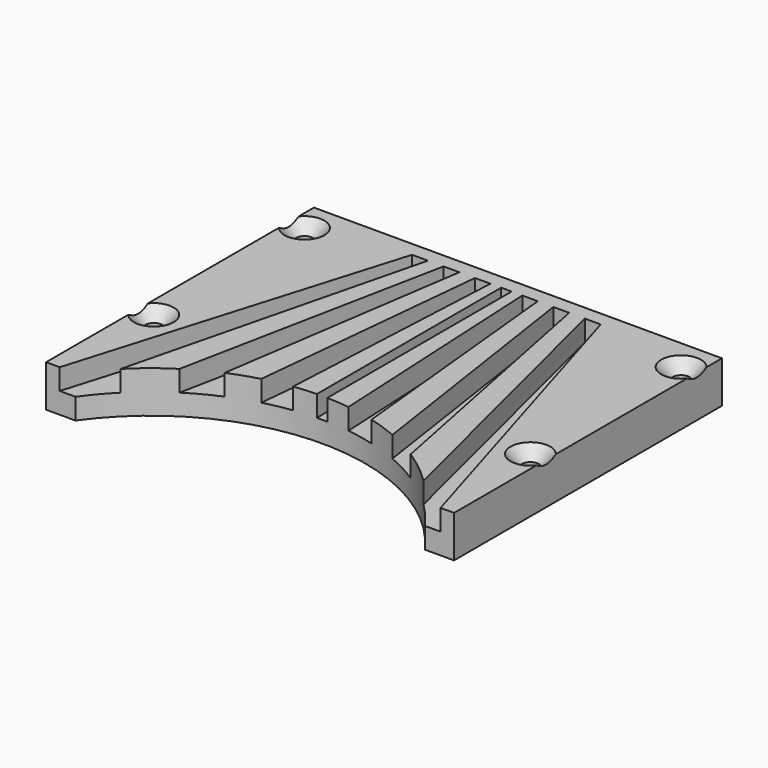
from build123d import *

# Parameters (mm, degrees)
F0_W           = 39
F0_H           = 40
F1_DEPTH       = 4
F4_DEPTH       = 25
F5_W           = 39
F5_H           = 7.9928017035
F6_DEPTH       = 25
F9_D           = 1.6
F9_CSINK_D     = 3.8
F9_CSINK_ANGLE = 90
F10_DEPTH      = 2
F12_DEPTH      = 0.9
F13_DEPTH      = 2


with BuildPart() as f1:
    # F0 (on Top) → F1 (new body)
    with BuildSketch(Plane.XY):
        Rectangle(F0_W, F0_H)
    extrude(amount=F1_DEPTH)

    # F3 (on face) → F4 (cut)
    with BuildSketch(Plane.XY.offset(4)):
        with BuildLine():
            Line((-16.7006288041, -20), (16.7006288041, -20))
            ThreePointArc((16.7006288041, -20), (0, -11.3886078894), (-16.7006288041, -20))
        make_face()
        with BuildLine():
            ThreePointArc((-16.7006288041, -20), (-6.2404771258, -51.4156774402), (20.5, -31.8886078894))
            ThreePointArc((20.5, -31.8886078894), (19.5270695508, -25.6481307636), (16.7006288041, -20))
            Line((16.7006288041, -20), (-16.7006288041, -20))
        make_face()
    extrude(amount=-F4_DEPTH, mode=Mode.SUBTRACT)

    # F5 (on face) → F6 (cut)
    with BuildSketch(Plane.XY.offset(4)):
        with Locations((0, 16.0035991482)):
            Rectangle(F5_W, F5_H)
    extrude(amount=-F6_DEPTH, mode=Mode.SUBTRACT)

    # F9 (through all)
    with Locations(Plane.XY.offset(4)):
        with Locations((18, 9), (18, -9), (-18, 9), (-18, -9)):
            CounterSinkHole(F9_D / 2, F9_CSINK_D / 2, counter_sink_angle=F9_CSINK_ANGLE)

    # F7 (on face) → F10 (cut)
    with BuildSketch(Plane.XY.offset(4)):
        with BuildLine():
            Line((0.5, 10.6266411021), (-0.5, 10.6266411021))
            Line((-0.5, 10.6266411021), (-0.5, -11.3947063575))
            ThreePointArc((-0.5, -11.3947063575), (0, -11.3886078894), (0.5, -11.3947063575))
            Line((0.5, -11.3947063575), (0.5, 10.6266411021))
        make_face()
        with BuildLine():
            ThreePointArc((-5.2656999319, -12.0764297096), (-3.9629214288, -11.7752975267), (-2.6432830651, -11.5597354505))
            Line((-2.6432830651, -11.5597354505), (-1.522443646, 10.6266411021))
            Line((-1.522443646, 10.6266411021), (-2.021334134, 10.6266411021))
            Line((-2.021334134, 10.6266411021), (-2.4928057101, 10.6266411021))
            Line((-2.4928057101, 10.6266411021), (-2.9997361505, 10.6266411021))
            Line((-2.9997361505, 10.6266411021), (-5.2656999319, -12.0764297096))
        make_face()
        with BuildLine():
            ThreePointArc((-11.0458529252, -14.6190064709), (-9.5659756043, -13.7573610835), (-8.0193476987, -13.0222340331))
            Line((-8.0193476987, -13.0222340331), (-4.491522759, 10.6266411021))
            Line((-4.491522759, 10.6266411021), (-4.9930326641, 10.6266411021))
            Line((-4.9930326641, 10.6266411021), (-5.5073648691, 10.6266411021))
            Line((-5.5073648691, 10.6266411021), (-6.005277995, 10.6266411021))
            Line((-6.005277995, 10.6266411021), (-11.0458529252, -14.6190064709))
        make_face()
        with BuildLine():
            ThreePointArc((-16.7006288041, -20), (-15.6412505167, -18.6371444882), (-14.4709725994, -17.3682445321))
            Line((-14.4709725994, -17.3682445321), (-7.4931742786, 10.6266411021))
            Line((-7.4931742786, 10.6266411021), (-7.993305102, 10.6266411021))
            Line((-7.993305102, 10.6266411021), (-8.507637307, 10.6266411021))
            Line((-8.507637307, 10.6266411021), (-9.0164762619, 10.6266411021))
            Line((-9.0164762619, 10.6266411021), (-18.1983038783, -20))
            Line((-18.1983038783, -20), (-17.6982320845, -20))
            Line((-17.6982320845, -20), (-16.7006288041, -20))
        make_face()
    extrude(amount=-F10_DEPTH, mode=Mode.SUBTRACT)

    # F11 (on face) → F12 (join)
    with BuildSketch(Plane(origin=(0, 0, 0), x_dir=(1, 0, 0), z_dir=(0, 0, -1))):
        with BuildLine():
            Line((1.5, 0), (6.9393398282, 5.4393398282))
            ThreePointArc((6.9393398282, 5.4393398282), (6.6141807012, 5.9259748515), (6.5, 6.5))
            ThreePointArc((6.5, 6.5), (5.9259748515, 6.6141807012), (5.4393398282, 6.9393398282))
            Line((5.4393398282, 6.9393398282), (0, 1.5))
            Line((0, 1.5), (1.5, 0))
        make_face()
        with BuildLine():
            ThreePointArc((6.5, 6.5), (6.6141807012, 5.9259748515), (6.9393398282, 5.4393398282))
            ThreePointArc((6.9393398282, 5.4393398282), (8.5740251485, 5.1141807012), (9.5, 6.5))
            ThreePointArc((9.5, 6.5), (9.0606601718, 7.5606601718), (8, 8))
            ThreePointArc((8, 8), (7.5606601718, 6.9393398282), (6.5, 6.5))
        make_face()
        with BuildLine():
            Line((6.5645856533, -5.0645856533), (1.5, 0))
            Line((1.5, 0), (0, -1.5))
            Line((0, -1.5), (5.4393398282, -6.9393398282))
            ThreePointArc((5.4393398282, -6.9393398282), (6.1413193654, -6.5435151211), (6.9468304687, -6.5680982812))
            ThreePointArc((6.9468304687, -6.5680982812), (6.5462462433, -5.8695943925), (6.5645856533, -5.0645856533))
        make_face()
        Polygon((0, -1.5), (1.5, 0), (0, 1.5), (-1.5, 0), align=None)
        with BuildLine():
            ThreePointArc((5.4393398282, 6.9393398282), (5.9259748515, 6.6141807012), (6.5, 6.5))
            ThreePointArc((6.5, 6.5), (6.9393398282, 7.5606601718), (8, 8))
            ThreePointArc((8, 8), (5.9259748515, 9.3858192988), (5.4393398282, 6.9393398282))
        make_face()
        with BuildLine():
            ThreePointArc((8, 8), (6.9393398282, 7.5606601718), (6.5, 6.5))
            ThreePointArc((6.5, 6.5), (7.5606601718, 6.9393398282), (8, 8))
        make_face()
        with BuildLine():
            Line((-5.4393398282, -6.9393398282), (0, -1.5))
            Line((0, -1.5), (-1.5, 0))
            Line((-1.5, 0), (-6.5645856533, -5.0645856533))
            ThreePointArc((-6.5645856533, -5.0645856533), (-5.7951926461, -5.6064457263), (-5.5, -6.5))
            ThreePointArc((-5.5, -6.5), (-5.5102000145, -6.6746310491), (-5.5406613378, -6.8468871126))
            ThreePointArc((-5.5406613378, -6.8468871126), (-5.4889432763, -6.8919547385), (-5.4393398282, -6.9393398282))
        make_face()
        with BuildLine():
            ThreePointArc((9.5, -5.5), (8.2200891637, -4.0162342638), (6.5645856533, -5.0645856533))
            ThreePointArc((6.5645856533, -5.0645856533), (6.5462462433, -5.8695943925), (6.9468304687, -6.5680982812))
            ThreePointArc((6.9468304687, -6.5680982812), (7.2717436331, -6.7137606114), (7.5531695313, -6.9319017188))
            ThreePointArc((7.5531695313, -6.9319017188), (8.8887503297, -6.7083554326), (9.5, -5.5))
        make_face()
        with BuildLine():
            Line((-1.5, 0), (0, 1.5))
            Line((0, 1.5), (-5.4393398282, 6.9393398282))
            ThreePointArc((-5.4393398282, 6.9393398282), (-5.9259748515, 6.6141807012), (-6.5, 6.5))
            ThreePointArc((-6.5, 6.5), (-6.6141807012, 5.9259748515), (-6.9393398282, 5.4393398282))
            Line((-6.9393398282, 5.4393398282), (-1.5, 0))
        make_face()
        with BuildLine():
            ThreePointArc((-5, -8), (-5.1141807012, -7.4259748515), (-5.4393398282, -6.9393398282))
            Line((-5.4393398282, -6.9393398282), (-5.6464466094, -7.1464466094))
            ThreePointArc((-5.6464466094, -7.1464466094), (-5.9393398282, -7.5606601718), (-6.3535533906, -7.8535533906))
            ThreePointArc((-6.3535533906, -7.8535533906), (-7.185794128, -7.9884490391), (-7.9593386622, -7.6531128874))
            ThreePointArc((-7.9593386622, -7.6531128874), (-6.6746310491, -9.4897999855), (-5, -8))
        make_face()
        with BuildLine():
            Line((-5.6464466094, -7.1464466094), (-5.4393398282, -6.9393398282))
            ThreePointArc((-5.4393398282, -6.9393398282), (-5.4889432763, -6.8919547385), (-5.5406613378, -6.8468871126))
            ThreePointArc((-5.5406613378, -6.8468871126), (-5.585601047, -6.9994753265), (-5.6464466094, -7.1464466094))
        make_face()
        with BuildLine():
            ThreePointArc((6.9468304687, -6.5680982812), (6.1413193654, -6.5435151211), (5.4393398282, -6.9393398282))
            ThreePointArc((5.4393398282, -6.9393398282), (5.9259748515, -9.3858192988), (8, -8))
            ThreePointArc((8, -8), (7.8837908615, -7.421102037), (7.5531695313, -6.9319017188))
            ThreePointArc((7.5531695313, -6.9319017188), (7.2282563669, -6.7862393886), (6.9468304687, -6.5680982812))
        make_face()
        with BuildLine():
            ThreePointArc((7.5531695313, -6.9319017188), (7.2717436331, -6.7137606114), (6.9468304687, -6.5680982812))
            ThreePointArc((6.9468304687, -6.5680982812), (7.2282563669, -6.7862393886), (7.5531695313, -6.9319017188))
        make_face()
        with BuildLine():
            ThreePointArc((-6.5, 6.5), (-5.9259748515, 6.6141807012), (-5.4393398282, 6.9393398282))
            ThreePointArc((-5.4393398282, 6.9393398282), (-5.1141807012, 7.4259748515), (-5, 8))
            ThreePointArc((-5, 8), (-6.5, 9.5), (-8, 8))
            ThreePointArc((-8, 8), (-6.9393398282, 7.5606601718), (-6.5, 6.5))
        make_face()
        with BuildLine():
            Line((-6.3535533906, -7.8535533906), (-5.6464466094, -7.1464466094))
            ThreePointArc((-5.6464466094, -7.1464466094), (-5.585601047, -6.9994753265), (-5.5406613378, -6.8468871126))
            ThreePointArc((-5.5406613378, -6.8468871126), (-6.974341649, -6.5769750529), (-7.9593386622, -7.6531128874))
            ThreePointArc((-7.9593386622, -7.6531128874), (-7.185794128, -7.9884490391), (-6.3535533906, -7.8535533906))
        make_face()
        with BuildLine():
            ThreePointArc((-7.9593386622, -7.6531128874), (-6.974341649, -6.5769750529), (-5.5406613378, -6.8468871126))
            ThreePointArc((-5.5406613378, -6.8468871126), (-5.5102000145, -6.6746310491), (-5.5, -6.5))
            ThreePointArc((-5.5, -6.5), (-5.7951926461, -5.6064457263), (-6.5645856533, -5.0645856533))
            ThreePointArc((-6.5645856533, -5.0645856533), (-8.3205084182, -5.7884822437), (-7.9593386622, -7.6531128874))
        make_face()
        with BuildLine():
            ThreePointArc((-8, 8), (-9.3858192988, 5.9259748515), (-6.9393398282, 5.4393398282))
            ThreePointArc((-6.9393398282, 5.4393398282), (-6.6141807012, 5.9259748515), (-6.5, 6.5))
            ThreePointArc((-6.5, 6.5), (-7.5606601718, 6.9393398282), (-8, 8))
        make_face()
        with BuildLine():
            ThreePointArc((-8, 8), (-7.5606601718, 6.9393398282), (-6.5, 6.5))
            ThreePointArc((-6.5, 6.5), (-6.9393398282, 7.5606601718), (-8, 8))
        make_face()
    extrude(amount=F12_DEPTH)

    # F7 (on face) → F13 (cut)
    with BuildSketch(Plane.XY.offset(4)):
        with BuildLine():
            Line((0.5, 10.6266411021), (-0.5, 10.6266411021))
            Line((-0.5, 10.6266411021), (-0.5, -11.3947063575))
            ThreePointArc((-0.5, -11.3947063575), (0, -11.3886078894), (0.5, -11.3947063575))
            Line((0.5, -11.3947063575), (0.5, 10.6266411021))
        make_face()
        with BuildLine():
            Line((1.522443646, 10.6266411021), (2.6491718308, -11.5605020108))
            ThreePointArc((2.6491718308, -11.5605020108), (3.9661171857, -11.7759274497), (5.2662566492, -12.0765776829))
            Line((5.2662566492, -12.0765776829), (2.9997361505, 10.6266411021))
            Line((2.9997361505, 10.6266411021), (2.498709131, 10.6266411021))
            Line((2.498709131, 10.6266411021), (2.0272377878, 10.6266411021))
            Line((2.0272377878, 10.6266411021), (1.522443646, 10.6266411021))
        make_face()
        with BuildLine():
            Line((4.491522759, 10.6266411021), (8.0269443273, -13.0254648648))
            ThreePointArc((8.0269443273, -13.0254648648), (9.5712306064, -13.7601345759), (11.048909782, -14.620962056))
            Line((11.048909782, -14.620962056), (6.005277995, 10.6266411021))
            Line((6.005277995, 10.6266411021), (5.4984204471, 10.6266411021))
            Line((5.4984204471, 10.6266411021), (4.9972091801, 10.6266411021))
            Line((4.9972091801, 10.6266411021), (4.491522759, 10.6266411021))
        make_face()
        with BuildLine():
            ThreePointArc((-16.7006288041, -20), (-15.6412505167, -18.6371444882), (-14.4709725994, -17.3682445321))
            Line((-14.4709725994, -17.3682445321), (-7.4931742786, 10.6266411021))
            Line((-7.4931742786, 10.6266411021), (-7.993305102, 10.6266411021))
            Line((-7.993305102, 10.6266411021), (-8.507637307, 10.6266411021))
            Line((-8.507637307, 10.6266411021), (-9.0164762619, 10.6266411021))
            Line((-9.0164762619, 10.6266411021), (-18.1983038783, -20))
            Line((-18.1983038783, -20), (-17.6982320845, -20))
            Line((-17.6982320845, -20), (-16.7006288041, -20))
        make_face()
        with BuildLine():
            Line((7.4931742786, 10.6266411021), (14.4761775715, -17.3734336598))
            ThreePointArc((14.4761775715, -17.3734336598), (15.6436257508, -18.6399485848), (16.7006288041, -20))
            Line((16.7006288041, -20), (17.7064798772, -20))
            Line((17.7064798772, -20), (18.2065498084, -20))
            Line((18.2065498084, -20), (9.0164762619, 10.6266411021))
            Line((9.0164762619, 10.6266411021), (8.5177253932, 10.6266411021))
            Line((8.5177253932, 10.6266411021), (7.9971281812, 10.6266411021))
            Line((7.9971281812, 10.6266411021), (7.4931742786, 10.6266411021))
        make_face()
    extrude(amount=-F13_DEPTH, mode=Mode.SUBTRACT)


solid = f1.part
